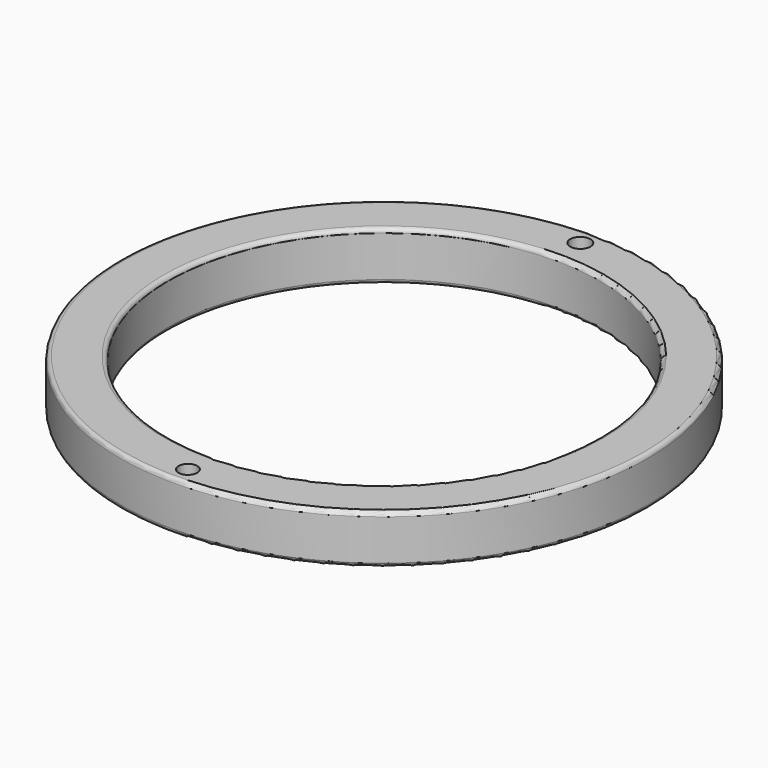
from build123d import *

# Parameters (mm, degrees)
F0_R     = 31.75
F0_R_2   = 1.125
F0_R_3   = 26
F0_R_4   = 1.225
F1_DEPTH = 5
F2_DEPTH = 5.9
F3_R     = 0.5
F4_R     = 0.5


with BuildPart() as f1:
    # F0 (on Top) → F1 (new body)
    with BuildSketch(Plane.XY):
        Circle(F0_R)
        with Locations((0, -29.5)):
            Circle(F0_R_2, mode=Mode.SUBTRACT)
        Circle(F0_R_3, mode=Mode.SUBTRACT)
        with Locations((0, 29.5)):
            Circle(F0_R_4, mode=Mode.SUBTRACT)
    extrude(amount=F1_DEPTH)

    # F0 (on Top) → F2 (join)
    with BuildSketch(Plane.XY):
        Circle(F0_R)
        with Locations((0, -29.5)):
            Circle(F0_R_2, mode=Mode.SUBTRACT)
        Circle(F0_R_3, mode=Mode.SUBTRACT)
        with Locations((0, 29.5)):
            Circle(F0_R_4, mode=Mode.SUBTRACT)
    extrude(amount=F2_DEPTH)

    # F3
    f3_edges = [f1.edges().sort_by_distance(p)[0] for p in [
        (-26, 0, 0),
        (-31.75, 0, 0),
        (-31.75, 0, 5.9),
    ]]
    fillet(f3_edges, radius=F3_R)

    # F4
    f4_edges = [f1.edges().sort_by_distance(p)[0] for p in [
        (-26, 0, 5.9),
        (-31.75, 0, 5.4),
    ]]
    fillet(f4_edges, radius=F4_R)


solid = f1.part
